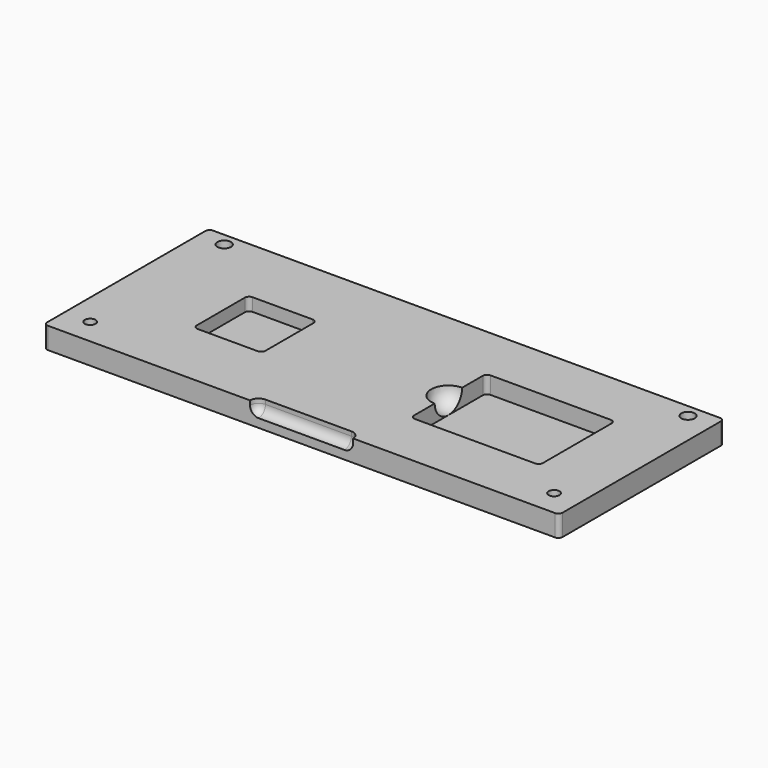
from build123d import *

# Parameters (mm, degrees)
F0_W      = 381
F0_H      = 152.4
F1_DEPTH  = 15.875
F3_DEPTH  = 9.525
F4_DEPTH  = 12.7
F5_R      = 3.175
F6_R      = 4
F7_DEPTH  = 5
F8_W      = 76.2
F8_H      = 9.525
F9_DEPTH  = 6.35
F10_R     = 6.34999
F11_R     = 5
F12_DEPTH = 15
F13_R     = 3.175


# Not quite as in the source:
# - a fillet or chamfer is up to 0.001 mm smaller than in the source, because OpenCascade refuses the exact size
# - ends of sketch curves that miss each other by under 0.0002 mm in the source are joined


with BuildPart() as f1:
    # F0 (on Top) → F1 (new body)
    with BuildSketch(Plane.XY):
        Rectangle(F0_W, F0_H)
    extrude(amount=-F1_DEPTH)

    # F2 (on face) → F3 (cut)
    with BuildSketch(Plane.XY):
        Polygon((-69.85, -25.4), (-69.85, 0), (-69.85, 25.4), (-120.65, 25.4), (-120.65, -25.4), align=None)
    extrude(amount=-F3_DEPTH, mode=Mode.SUBTRACT)

    # F2 (on face) → F4 (cut)
    with BuildSketch(Plane.XY):
        Polygon((47.625, 0), (47.625, -34.925), (142.875, -34.925), (142.875, 34.925), (47.625, 34.925), align=None)
    extrude(amount=-F4_DEPTH, mode=Mode.SUBTRACT)

    # F5
    f5_edges = [f1.edges().sort_by_distance(p)[0] for p in [
        (-69.85, 25.4, -4.7625),
        (142.875, 34.925, -6.35),
        (-69.85, -25.4, -4.7625),
        (142.875, -34.925, -6.35),
        (-120.65, -25.4, -4.7625),
        (47.625, -34.925, -6.35),
        (47.625, 34.925, -6.35),
        (-120.65, 25.4, -4.7625),
    ]]
    fillet(f5_edges, radius=F5_R)

    # F6 (on face) → F7 (cut)
    with BuildSketch(Plane.XY):
        with Locations((-171.4581174665, -57.1581174665)):
            Circle(F6_R)
        with Locations((171.4581174665, -57.1581174665)):
            Circle(F6_R)
    extrude(amount=-F7_DEPTH, mode=Mode.SUBTRACT)

    # F8 (on face) → F9 (cut)
    with BuildSketch(Plane.XZ.offset(76.2)):
        with Locations((0, -4.7625)):
            Rectangle(F8_W, F8_H)
    extrude(amount=-F9_DEPTH, mode=Mode.SUBTRACT)

    # F10 (radius 6.35 in the source; OpenCascade refuses exactly that, so slightly less here)
    f10_edges = [f1.edges().sort_by_distance(p)[0] for p in [
        (-38.1, -73.025, -9.525),
        (-38.1, -69.85, -4.7625),
        (0, -69.85, -9.525),
        (38.1, -73.025, -9.525),
        (38.1, -69.85, -4.7625),
    ]]
    fillet(f10_edges, radius=F10_R)

    # F11 (on face) → F12 (cut)
    with BuildSketch(Plane.XY):
        with Locations((-171.45, 66.675)):
            Circle(F11_R)
        with Locations((171.45, 66.675)):
            Circle(F11_R)
    extrude(amount=-F12_DEPTH, mode=Mode.SUBTRACT)

    # F13
    f13_edges = [f1.edges().sort_by_distance(p)[0] for p in [
        (-190.5, -76.2, -7.9375),
        (190.5, -76.2, -7.9375),
        (190.5, 76.2, -7.9375),
        (-190.5, 76.2, -7.9375),
    ]]
    fillet(f13_edges, radius=F13_R)

    # F14 (on face) → F15 (revolve, cut)
    with BuildSketch(Plane.XY):
        with BuildLine():
            Line((47.625, -12.7), (47.625, 12.7))
            ThreePointArc((47.625, 12.7), (34.925, 1.535e-07), (47.625, -12.7))
        make_face()
    revolve(axis=Axis((47.625, 0, 0), (0, -1, 0)), mode=Mode.SUBTRACT)


solid = f1.part
